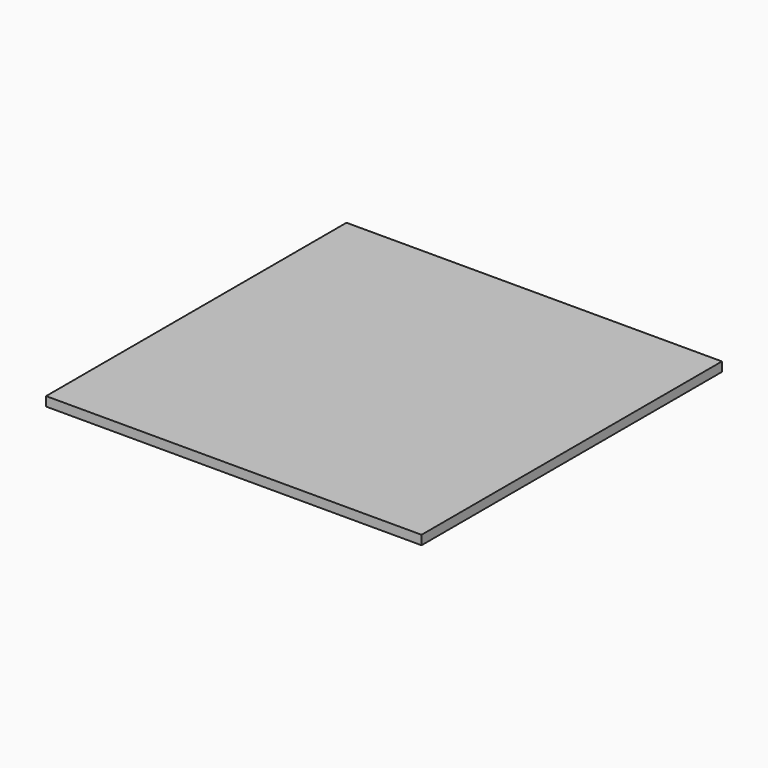
from build123d import *

# Parameters (mm, degrees)
F0_W     = 650
F0_H     = 650
F0_R     = 4
F1_DEPTH = 16
F2_DEPTH = 10


# Not quite as in the source:
# - a pattern or mirror of a feature is missing from the dataset's text; its kind, count and spacing are read off the source's solid


with BuildPart() as f1:
    # F0 (on Top) → F1 (new body)
    with BuildSketch(Plane.XY):
        Rectangle(F0_W, F0_H)
        with Locations((-315, -261)):
            Circle(F0_R, mode=Mode.SUBTRACT)
        with Locations((-315, -155.8)):
            Circle(F0_R, mode=Mode.SUBTRACT)
        with Locations((-315, -50.6)):
            Circle(F0_R, mode=Mode.SUBTRACT)
        with Locations((-315, 54.6)):
            Circle(F0_R, mode=Mode.SUBTRACT)
        with Locations((-315, 159.8)):
            Circle(F0_R, mode=Mode.SUBTRACT)
        with Locations((-315, 265)):
            Circle(F0_R, mode=Mode.SUBTRACT)
        with Locations((-315, 265)):
            Circle(F0_R)
        with Locations((-315, 159.8)):
            Circle(F0_R)
        with Locations((-315, 54.6)):
            Circle(F0_R)
        with Locations((-315, -50.6)):
            Circle(F0_R)
        with Locations((-315, -155.8)):
            Circle(F0_R)
        with Locations((-315, -261)):
            Circle(F0_R)
    extrude(amount=F1_DEPTH)

    # F0 (on Top) → F2 (cut)
    with BuildSketch(Plane.XY):
        with Locations((-315, 265)):
            Circle(F0_R)
        with Locations((-315, 159.8)):
            Circle(F0_R)
        with Locations((-315, 54.6)):
            Circle(F0_R)
        with Locations((-315, -50.6)):
            Circle(F0_R)
        with Locations((-315, -155.8)):
            Circle(F0_R)
        with Locations((-315, -261)):
            Circle(F0_R)
    f2 = extrude(amount=F2_DEPTH, mode=Mode.SUBTRACT)

    # F2_copies: F2 across plane
    add(f2.mirror(Plane(origin=(0, 0, 0), x_dir=(0, 0, 1), z_dir=(1, 0, 0))), mode=Mode.SUBTRACT)


solid = f1.part
